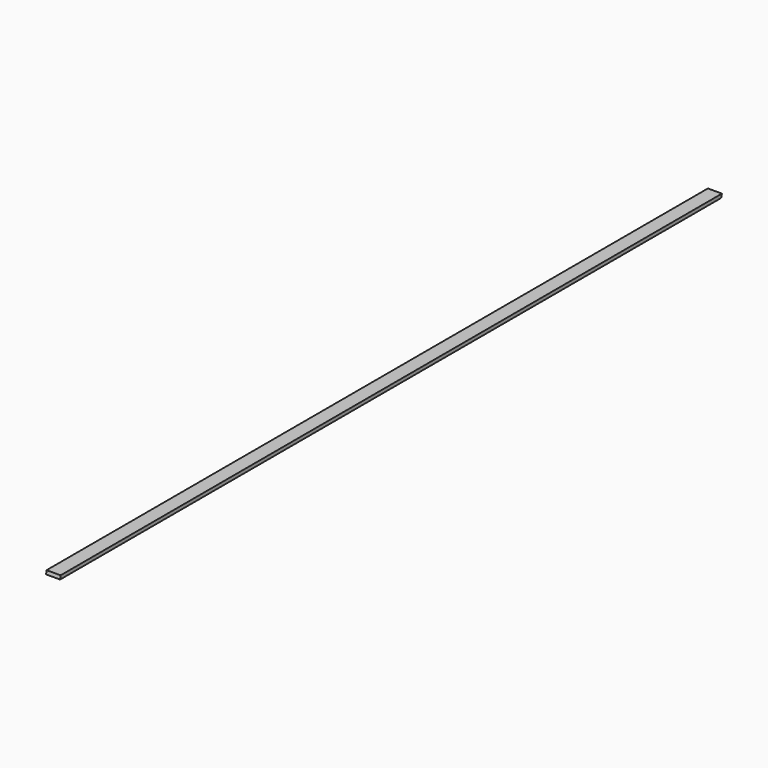
from build123d import *

# Parameters (mm, degrees)
F0_W     = 25.4
F0_H     = 1500.7336
F1_DEPTH = 6.35
F3_DEPTH = 25.401


# Not quite as in the source:
# - a feature names something its author has since deleted; it is built from what else it names


with BuildPart() as f1:
    # F0 (on Top) → F1 (new body)
    with BuildSketch(Plane.XY):
        with Locations((12.7, 750.3668)):
            Rectangle(F0_W, F0_H)
    extrude(amount=F1_DEPTH)

    # F2 (on face) → F3 (cut, through all)
    with BuildSketch(Plane.YZ.offset(25.4)):
        Polygon((1.1196763275, 6.35), (0, 6.35), (0, 0), align=None)
        Polygon((1500.7336, 6.35), (1499.0321226281, 0), (1500.7336, 0), align=None)
    extrude(amount=-F3_DEPTH, mode=Mode.SUBTRACT)


solid = f1.part
